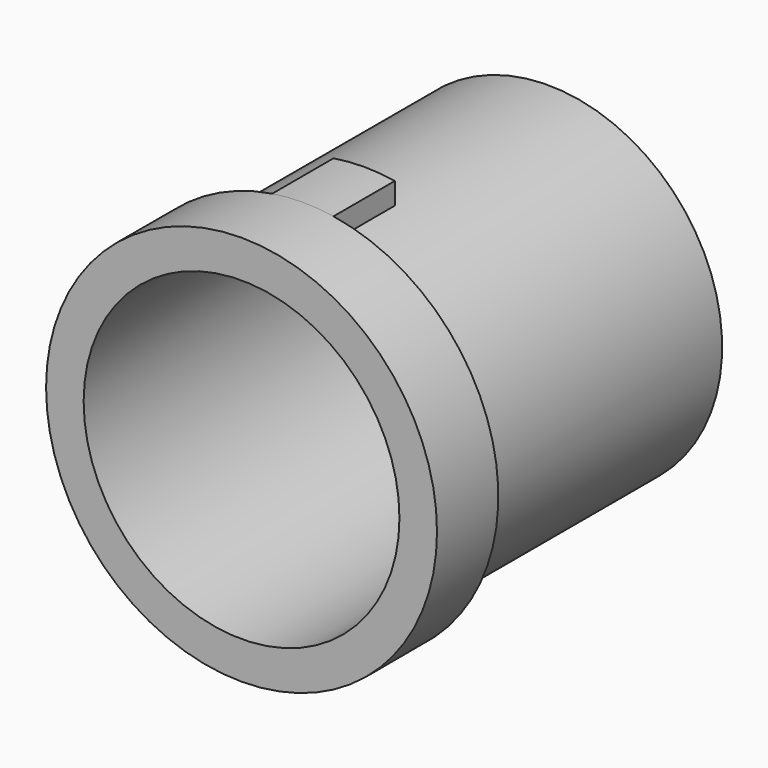
from build123d import *

# Parameters (mm, degrees)
F0_R         = 10.3
F1_DEPTH     = 9
F3_R         = 3.1
F4_DEPTH     = 9.001
F6_DEPTH     = 1.8
F7_T4_ANGLE  = 359.64
F7_S5_R      = 3.1
F7_T6_DEPTH  = 5
F7_T10_ANGLE = 359.64
F7_S11_R     = 3.1
F7_T12_DEPTH = 5
F7_T16_ANGLE = 359.64
F7_S17_R     = 3.1
F7_T18_DEPTH = 5
F9_R         = 12.75
F10_DEPTH    = 25
F11_R        = 3.1
F12_DEPTH    = 34.0010001
F13_R        = 12.75
F13_R_2      = 11.35
F14_DEPTH    = 20
F16_DEPTH    = 5
F17_R        = 10.3
F18_DEPTH    = 34.0010001
F20_START    = -5
F20_DEPTH    = 5


# Not quite as in the source:
# - a fillet or chamfer that OpenCascade refuses, or shapes differently, is made with other operations: its cross-section is extruded or revolved along the edge and cut away or added


with BuildPart() as f1:
    # F0 (on Front) → F1 (new body)
    with BuildSketch(Plane.XZ):
        Circle(F0_R)
    extrude(amount=F1_DEPTH)

    # F3 (on face) → F4 (cut, through all)
    with BuildSketch(Plane.XZ.offset(9)):
        Circle(F3_R)
    extrude(amount=-F4_DEPTH, mode=Mode.SUBTRACT)

    # F5 (on face) → F6 (cut)
    with BuildSketch(Plane.XZ.offset(9)):
        with BuildLine():
            ThreePointArc((-3.0819681678, 0.333874546), (-2.6846787517, 1.55), (-1.8301279224, 2.502125454))
            ThreePointArc((-1.8301279224, 2.502125454), (-6.4951905284, 3.75), (-3.0819681678, 0.333874546))
        make_face()
        with BuildLine():
            ThreePointArc((6.8301270189, 2.5), (4.331189746, 4.9999997741), (1.8301279224, 2.502125454))
            ThreePointArc((1.8301279224, 2.502125454), (2.6846787517, 1.55), (3.0819681678, 0.333874546))
            ThreePointArc((3.0819681678, 0.333874546), (5.5810472546, 0.3354680497), (6.8301270189, 2.5))
        make_face()
        with BuildLine():
            ThreePointArc((1.2518402454, -2.836), (0, -3.1), (-1.2518402454, -2.836))
            ThreePointArc((-1.2518402454, -2.836), (-1.2490795384, -7.1655946774), (2.5, -5))
            ThreePointArc((2.5, -5), (2.1655946774, -3.7509204616), (1.2518402454, -2.836))
        make_face()
    extrude(amount=-F6_DEPTH, mode=Mode.SUBTRACT)

    # F7: fillet of radius 1 on 3 edges, made by hand


with BuildPart() as f7_tool2:
    # F7_s3 → F7_t4 (revolve)
    with BuildSketch(Plane(origin=(0.0078111935, 0, 0.0136280797), x_dir=(0, 1, 0), z_dir=(-0.497276838, 0, -0.8675919239))):
        with BuildLine():
            ThreePointArc((-8.2, -2.499975326), (-7.4928932188, -2.7928685448), (-7.2, -3.499975326))
            Line((-7.2, -3.499975326), (-7.18, -3.499975326))
            Line((-7.18, -3.499975326), (-7.18, -2.479975326))
            Line((-7.18, -2.479975326), (-8.2, -2.479975326))
            Line((-8.2, -2.479975326), (-8.2, -2.499975326))
        make_face()
    revolve(axis=Axis((-4.3301270189, -7.2, 2.5), (0, -1, 0)), revolution_arc=F7_T4_ANGLE)

    # F7_s5 → F7_t6 (cut, symmetric)
    with BuildSketch(Plane.XZ.offset(7.7)):
        Circle(F7_S5_R)
    extrude(amount=F7_T6_DEPTH, both=True, mode=Mode.SUBTRACT)


with BuildPart() as f1_1:
    add(f1.part)

    # F7_t1: union F7_tool2
    add(f7_tool2.part)


with BuildPart() as f7_tool8:
    # F7_s9 → F7_t10 (revolve)
    with BuildSketch(Plane(origin=(0.0078966665, 0, -0.0135787318), x_dir=(0, 1, 0), z_dir=(-0.5027182272, 0, 0.8644503364))):
        with BuildLine():
            ThreePointArc((-8.2, -2.499975326), (-7.4928932188, -2.7928685448), (-7.2, -3.499975326))
            Line((-7.2, -3.499975326), (-7.18, -3.499975326))
            Line((-7.18, -3.499975326), (-7.18, -2.479975326))
            Line((-7.18, -2.479975326), (-8.2, -2.479975326))
            Line((-8.2, -2.479975326), (-8.2, -2.499975326))
        make_face()
    revolve(axis=Axis((4.3301270189, -7.2, 2.5), (0, -1, 0)), revolution_arc=F7_T10_ANGLE)

    # F7_s11 → F7_t12 (cut, symmetric)
    with BuildSketch(Plane.XZ.offset(7.7)):
        Circle(F7_S11_R)
    extrude(amount=F7_T12_DEPTH, both=True, mode=Mode.SUBTRACT)


with BuildPart() as f1_2:
    add(f1_1.part)

    # F7_t7: union F7_tool8
    add(f7_tool8.part)


with BuildPart() as f7_tool14:
    # F7_s15 → F7_t16 (revolve)
    with BuildSketch(Plane(origin=(-0.0157078599, 0, -4.93479e-05), x_dir=(0, 1, 0), z_dir=(0.9999950652, 0, 0.0031415875))):
        with BuildLine():
            ThreePointArc((-8.2, -2.499975326), (-7.4928932188, -2.7928685448), (-7.2, -3.499975326))
            Line((-7.2, -3.499975326), (-7.18, -3.499975326))
            Line((-7.18, -3.499975326), (-7.18, -2.479975326))
            Line((-7.18, -2.479975326), (-8.2, -2.479975326))
            Line((-8.2, -2.479975326), (-8.2, -2.499975326))
        make_face()
    revolve(axis=Axis((0, -7.2, -5), (0, -1, 0)), revolution_arc=F7_T16_ANGLE)

    # F7_s17 → F7_t18 (cut, symmetric)
    with BuildSketch(Plane.XZ.offset(7.7)):
        Circle(F7_S17_R)
    extrude(amount=F7_T18_DEPTH, both=True, mode=Mode.SUBTRACT)


with BuildPart() as f1_3:
    add(f1_2.part)

    # F7_t13: union F7_tool14
    add(f7_tool14.part)

    # F9 (on offset) → F10 (join)
    with BuildSketch(Plane(origin=(0, 0, 0), x_dir=(-1, 0, 0), z_dir=(0, 1, 0))):
        Circle(F9_R)
    extrude(amount=F10_DEPTH)

    # F11 (on face) → F12 (cut, through all)
    with BuildSketch(Plane(origin=(0, 25, 0), x_dir=(-1, 0, 0), z_dir=(0, 1, 0))):
        Circle(F11_R)
    extrude(amount=-F12_DEPTH, mode=Mode.SUBTRACT)

    # F13 (on face) → F14 (cut)
    with BuildSketch(Plane(origin=(0, 25, 0), x_dir=(-1, 0, 0), z_dir=(0, 1, 0))):
        Circle(F13_R)
        Circle(F13_R_2, mode=Mode.SUBTRACT)
    extrude(amount=-F14_DEPTH, mode=Mode.SUBTRACT)

    # F15 (on face) → F16 (join)
    with BuildSketch(Plane(origin=(0, 5, 0), x_dir=(-1, 0, 0), z_dir=(0, 1, 0))):
        with BuildLine():
            ThreePointArc((2, 12.5921602595), (0, 12.75), (-2, 12.5921602595))
            Line((-2, 12.5921602595), (-2, 11.1723990262))
            ThreePointArc((-2, 11.1723990262), (0, 11.35), (2, 11.1723990262))
            Line((2, 11.1723990262), (2, 12.5921602595))
        make_face()
        with BuildLine():
            ThreePointArc((2, -11.1723990262), (0, -11.35), (-2, -11.1723990262))
            Line((-2, -11.1723990262), (-2, -12.5921602595))
            ThreePointArc((-2, -12.5921602595), (0, -12.75), (2, -12.5921602595))
            Line((2, -12.5921602595), (2, -11.1723990262))
        make_face()
    extrude(amount=F16_DEPTH)

    # F17 (on face) → F18 (cut, through all)
    with BuildSketch(Plane.XZ.offset(9)):
        Circle(F17_R)
    extrude(amount=-F18_DEPTH, mode=Mode.SUBTRACT)

    # F19 (on face) → F20 (join)
    with BuildSketch(Plane(origin=(0, 25, 0), x_dir=(-1, 0, 0), z_dir=(0, 1, 0)).offset(F20_START)):
        with BuildLine():
            Line((-7.5, 0), (-10.3, 0))
            ThreePointArc((-10.3, 0), (-9.5744451536, -3.7973675092), (-7.5, -7.0597450379))
            Line((-7.5, -7.0597450379), (-7.5, 0))
        make_face()
    extrude(amount=-F20_DEPTH)


solid = f1_3.part
